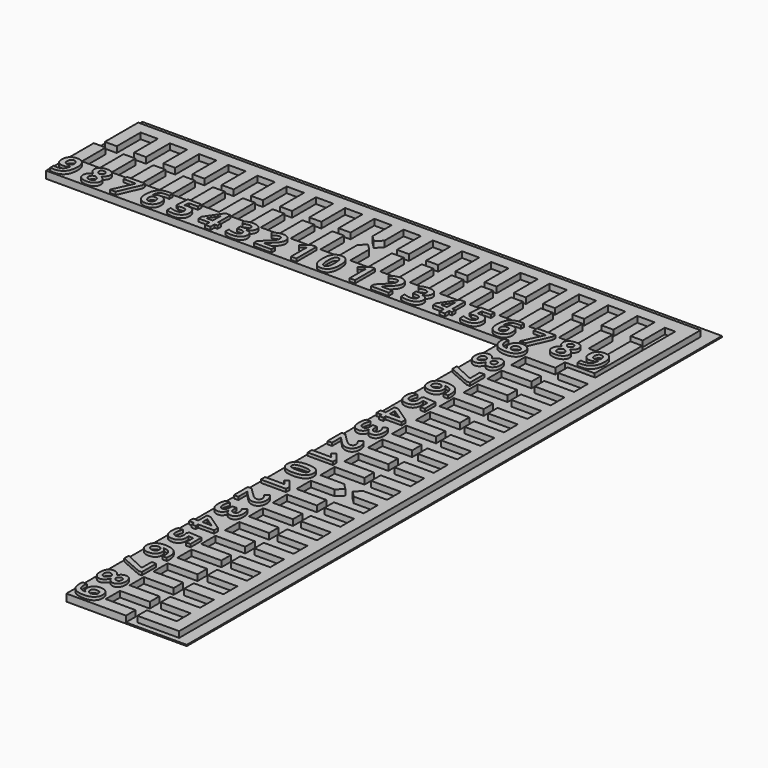
from build123d import *

# Parameters (mm, degrees)
F0_W         = 2
F0_H         = 5
F1_DEPTH     = 1
F2_W         = 2
F2_H         = 5
F3_DEPTH     = 1
F6_TEXT_SIZE = 5.9155665401
F7_DEPTH     = 0.5
F8_SIZE      = 0.99999
F8_2_SIZE    = 0.99999
F9_ANGLE     = 90
F10_ANGLE    = 90
F13_DEPTH    = 1
F15_DEPTH    = 0.2


# Not quite as in the source:
# - a fillet or chamfer is up to 0.001 mm smaller than in the source, because OpenCascade refuses the exact size
# - Text() gives the source's letters only with a copy of the font that has no kerning and outlines rounded to 1/6400 em; it was checked with that copy


with BuildPart() as f1:
    # F0 (on Top) → F1 (new body)
    with BuildSketch(Plane.XY):
        with Locations((0, 2.5)):
            Rectangle(F0_W, F0_H)
        Polygon((1, 0), (-1, 0), (-4, 0), (-6, 0), (-9, 0), (-11, 0), (-14, 0), (-16, 0), (-19, 0), (-21, 0), (-24, 0), (-26, 0), (-29, 0), (-31, 0), (-34, 0), (-36, 0), (-39, 0), (-41, 0), (-44, 0), (-46, 0), (-46, -5), (46, -5), (46, 0), (44, 0), (41, 0), (39, 0), (36, 0), (34, 0), (31, 0), (29, 0), (26, 0), (24, 0), (21, 0), (19, 0), (16, 0), (14, 0), (11, 0), (9, 0), (6, 0), (4, 0), align=None)
        with Locations((-5, 2.5)):
            Rectangle(F0_W, F0_H)
        with Locations((5, 2.5)):
            Rectangle(F0_W, F0_H)
        with Locations((-10, 2.5)):
            Rectangle(F0_W, F0_H)
        with Locations((10, 2.5)):
            Rectangle(F0_W, F0_H)
        with Locations((-15, 2.5)):
            Rectangle(F0_W, F0_H)
        with Locations((15, 2.5)):
            Rectangle(F0_W, F0_H)
        with Locations((-20, 2.5)):
            Rectangle(F0_W, F0_H)
        with Locations((20, 2.5)):
            Rectangle(F0_W, F0_H)
        with Locations((-25, 2.5)):
            Rectangle(F0_W, F0_H)
        with Locations((25, 2.5)):
            Rectangle(F0_W, F0_H)
        with Locations((-30, 2.5)):
            Rectangle(F0_W, F0_H)
        with Locations((30, 2.5)):
            Rectangle(F0_W, F0_H)
        with Locations((-35, 2.5)):
            Rectangle(F0_W, F0_H)
        with Locations((35, 2.5)):
            Rectangle(F0_W, F0_H)
        with Locations((-40, 2.5)):
            Rectangle(F0_W, F0_H)
        with Locations((40, 2.5)):
            Rectangle(F0_W, F0_H)
        with Locations((-45, 2.5)):
            Rectangle(F0_W, F0_H)
        with Locations((45, 2.5)):
            Rectangle(F0_W, F0_H)
    extrude(amount=F1_DEPTH)

    # F6 (on face) → F7 (join)
    with BuildSketch(Plane.XY.offset(1)):
        with Locations((-46, -4.7242937544)):
            Text('9 8 7 6 5 4 3 2 1 0 1 2 3 4 5 6 7 8 9', F6_TEXT_SIZE, font='Open Sans', font_style=FontStyle.BOLD, text_align=(TextAlign.LEFT, TextAlign.BOTTOM))
    extrude(amount=F7_DEPTH)

    # F8 (size 1 in the source; OpenCascade refuses exactly that, so slightly less here)
    f8_edges = [f1.edges().sort_by_distance(p)[0] for p in [
        (1, 5, 0.5),
        (-1, 5, 0.5),
    ]]
    chamfer(f8_edges, length=F8_SIZE)


with BuildPart() as f3:
    # F2 (on Top) → F3 (new body)
    with BuildSketch(Plane.XY):
        with Locations((0, -8.6960415205)):
            Rectangle(F2_W, F2_H)
        Polygon((1, -11.1960415205), (-1, -11.1960415205), (-3.9, -11.1960415205), (-5.9, -11.1960415205), (-8.8, -11.1960415205), (-10.8, -11.1960415205), (-13.7, -11.1960415205), (-15.7, -11.1960415205), (-18.6, -11.1960415205), (-20.6, -11.1960415205), (-23.5, -11.1960415205), (-25.5, -11.1960415205), (-28.4, -11.1960415205), (-30.4, -11.1960415205), (-33.3, -11.1960415205), (-35.3, -11.1960415205), (-38.2, -11.1960415205), (-40.2, -11.1960415205), (-43.1, -11.1960415205), (-45.1, -11.1960415205), (-45.1, -13.1960415205), (45.1, -13.1960415205), (45.1, -11.1960415205), (43.1, -11.1960415205), (40.2, -11.1960415205), (38.2, -11.1960415205), (35.3, -11.1960415205), (33.3, -11.1960415205), (30.4, -11.1960415205), (28.4, -11.1960415205), (25.5, -11.1960415205), (23.5, -11.1960415205), (20.6, -11.1960415205), (18.6, -11.1960415205), (15.7, -11.1960415205), (13.7, -11.1960415205), (10.8, -11.1960415205), (8.8, -11.1960415205), (5.9, -11.1960415205), (3.9, -11.1960415205), align=None)
        with Locations((-4.9, -8.6960415205)):
            Rectangle(F2_W, F2_H)
        with Locations((4.9, -8.6960415205)):
            Rectangle(F2_W, F2_H)
        with Locations((-9.8, -8.6960415205)):
            Rectangle(F2_W, F2_H)
        with Locations((9.8, -8.6960415205)):
            Rectangle(F2_W, F2_H)
        with Locations((-14.7, -8.6960415205)):
            Rectangle(F2_W, F2_H)
        with Locations((14.7, -8.6960415205)):
            Rectangle(F2_W, F2_H)
        with Locations((-19.6, -8.6960415205)):
            Rectangle(F2_W, F2_H)
        with Locations((19.6, -8.6960415205)):
            Rectangle(F2_W, F2_H)
        with Locations((-24.5, -8.6960415205)):
            Rectangle(F2_W, F2_H)
        with Locations((24.5, -8.6960415205)):
            Rectangle(F2_W, F2_H)
        with Locations((-29.4, -8.6960415205)):
            Rectangle(F2_W, F2_H)
        with Locations((29.4, -8.6960415205)):
            Rectangle(F2_W, F2_H)
        with Locations((-34.3, -8.6960415205)):
            Rectangle(F2_W, F2_H)
        with Locations((34.3, -8.6960415205)):
            Rectangle(F2_W, F2_H)
        with Locations((-39.2, -8.6960415205)):
            Rectangle(F2_W, F2_H)
        with Locations((39.2, -8.6960415205)):
            Rectangle(F2_W, F2_H)
        with Locations((-44.1, -8.6960415205)):
            Rectangle(F2_W, F2_H)
        with Locations((44.1, -8.6960415205)):
            Rectangle(F2_W, F2_H)
    extrude(amount=F3_DEPTH)


with BuildPart() as f4_1:
    # F4: instance of F3
    add(f3.part.mirror(Plane.XZ))

    # F8#2 (size 1 in the source; OpenCascade refuses exactly that, so slightly less here)
    f8_2_edges = [f4_1.edges().sort_by_distance(p)[0] for p in [
        (-1, 6.196042, 0.5),
        (1, 6.196042, 0.5),
    ]]
    chamfer(f8_2_edges, length=F8_2_SIZE)


with BuildPart() as f9_1:
    # F9: copy of F1
    add(f1.part.rotate(Axis((-46, -5, 0.5), (0, 0, -1)), F9_ANGLE))


with BuildPart() as f10_1:
    # F10: copy of F4_1
    add(f4_1.part.rotate(Axis((-46, -5, 0.5), (0, 0, -1)), F10_ANGLE))


with BuildPart() as f9_1_1:
    # F11: moved
    add(f9_1.part.moved(Location((77, 0, 0))))


with BuildPart() as f10_1_1:
    # F11: moved
    add(f10_1.part.moved(Location((77, 0, 0))))


with BuildPart() as f4_1_1:
    add(f4_1.part)

    add(f10_1_1.part)  # F13 merges F10_1
    # F12 (on Top) → F13 (join)
    with BuildSketch(Plane.XY):
        Polygon((46.8474816119, -5.9), (49.1960415205, -5.9), (49.1960415205, 13.1960415205), (45.1, 13.1960415205), (45.1, 10.8474816119), (46.8474816119, 10.8474816119), align=None)
    extrude(amount=F13_DEPTH)


with BuildPart() as f1_1:
    add(f1.part)

    add(f9_1_1.part)  # F15 merges F9_1
    # F14 (on Top) → F15 (join)
    with BuildSketch(Plane.XY):
        Polygon((-46, 15.1960415205), (-46, -5), (31, -5), (31, -97), (51.1960415205, -97), (51.1960415205, 15.1960415205), align=None)
    extrude(amount=-F15_DEPTH)


solid = Compound([f4_1_1.part, f1_1.part])
